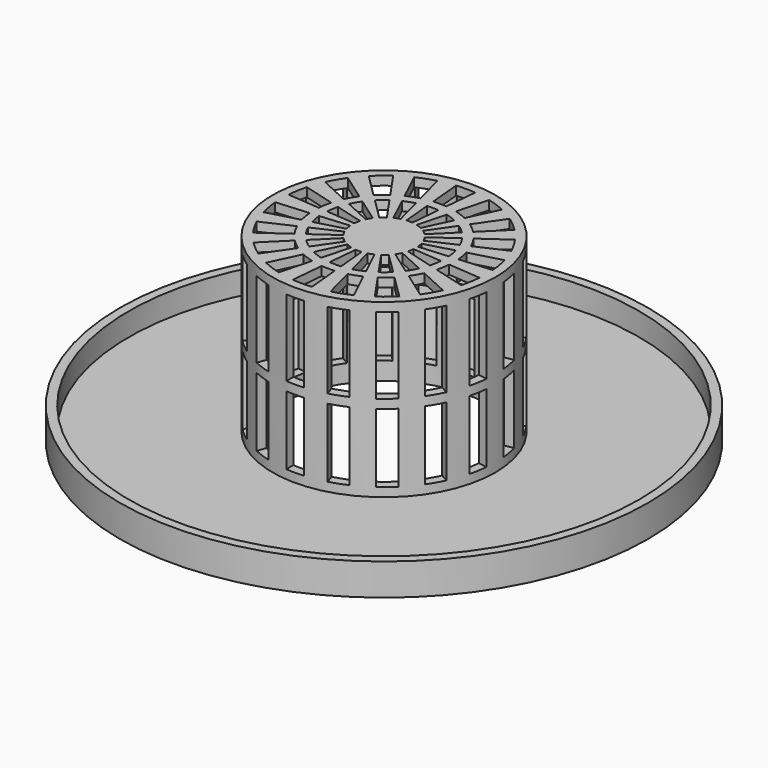
from build123d import *
from build123d import SkipClean  # not in build123d's __all__

# Parameters (mm, degrees)
F0_R             = 52.705
F1_DEPTH         = 6.35
F2_T             = -1.778
F3_R             = 22.225
F4_DEPTH         = 34.29
F5_W             = 3.556
F5_H             = 15.24
F5_H_2           = 13.716
F6_DEPTH         = 25.4
F6_COPIES_COUNT  = 9
F6_COPIES_ANGLE  = 160
F7_R             = 20.447
F8_DEPTH         = 34.29
F10_DEPTH        = 25.4
F10_COPIES_COUNT = 18


# Not quite as in the source:
# - after a boolean that leaves OpenCascade's solid faulty, fix() repairs it
# - a pattern or mirror of a feature is missing from the dataset's text; its kind, count and spacing are read off the source's solid


with BuildPart() as f1:
    # F0 (on Top) → F1 (new body)
    with BuildSketch(Plane.XY):
        Circle(F0_R)
    extrude(amount=F1_DEPTH)

    # F2
    f2_openings = [f1.faces().sort_by_distance(p)[0] for p in [
        (0, 0, 6.35),
    ]]
    offset(amount=F2_T, openings=f2_openings)

    # F3 (on face) → F4 (join)
    with BuildSketch(Plane.XY.offset(1.778)):
        Circle(F3_R)
    extrude(amount=F4_DEPTH)

    # F5 (on Front) → F6 (cut, symmetric)
    with BuildSketch(Plane.XZ):
        with Locations((0, 26.67)):
            Rectangle(F5_W, F5_H)
        with Locations((0, 10.414)):
            Rectangle(F5_W, F5_H_2)
    f6 = extrude(amount=F6_DEPTH, both=True, mode=Mode.SUBTRACT)

    # F6_copies: F6 ×9 about axis
    f6_copies_axis = Axis((0, 0, 0), (0, 0, -1))
    for i in range(1, F6_COPIES_COUNT):
        add(f6.rotate(f6_copies_axis, i * F6_COPIES_ANGLE / (F6_COPIES_COUNT - 1)), clean=False, mode=Mode.SUBTRACT)

    # F7 (on face) → F8 (cut)
    with BuildSketch(Plane(origin=(0, 0, 0), x_dir=(1, 0, 0), z_dir=(0, 0, -1))):
        Circle(F7_R)
    extrude(amount=-F8_DEPTH, mode=Mode.SUBTRACT)

    # F9 (on face) → F10 (cut)
    with BuildSketch(Plane.XY.offset(36.068)):
        with BuildLine():
            Line((-1.3038666667, -13.9090197971), (-1.9083866667, -20.3577471575))
            ThreePointArc((-1.9083866667, -20.3577471575), (0, -20.447), (1.9083866667, -20.3577471575))
            Line((1.9083866667, -20.3577471575), (1.3038666667, -13.9090197971))
            ThreePointArc((1.3038666667, -13.9090197971), (0, -13.97), (-1.3038666667, -13.9090197971))
        make_face()
        with BuildLine():
            Line((-0.5926666667, -6.3222817259), (-1.13792, -12.1387809138))
            ThreePointArc((-1.13792, -12.1387809138), (0, -12.192), (1.13792, -12.1387809138))
            Line((1.13792, -12.1387809138), (0.5926666667, -6.3222817259))
            ThreePointArc((0.5926666667, -6.3222817259), (0, -6.35), (-0.5926666667, -6.3222817259))
        make_face()
    f10 = extrude(amount=-F10_DEPTH, mode=Mode.SUBTRACT)

    # F10_copies: F10 ×18 about axis
    f10_copies_axis = Axis((0, 0, 0), (0, 0, 1))
    with SkipClean():  # cleaning this boolean's faces spoils the solid; the shape is the same uncleaned
        for i in range(1, F10_COPIES_COUNT):
            add(f10.rotate(f10_copies_axis, i * 360 / F10_COPIES_COUNT), clean=False, mode=Mode.SUBTRACT)

    add(f1.part.fix(), mode=Mode.REPLACE)


solid = f1.part
